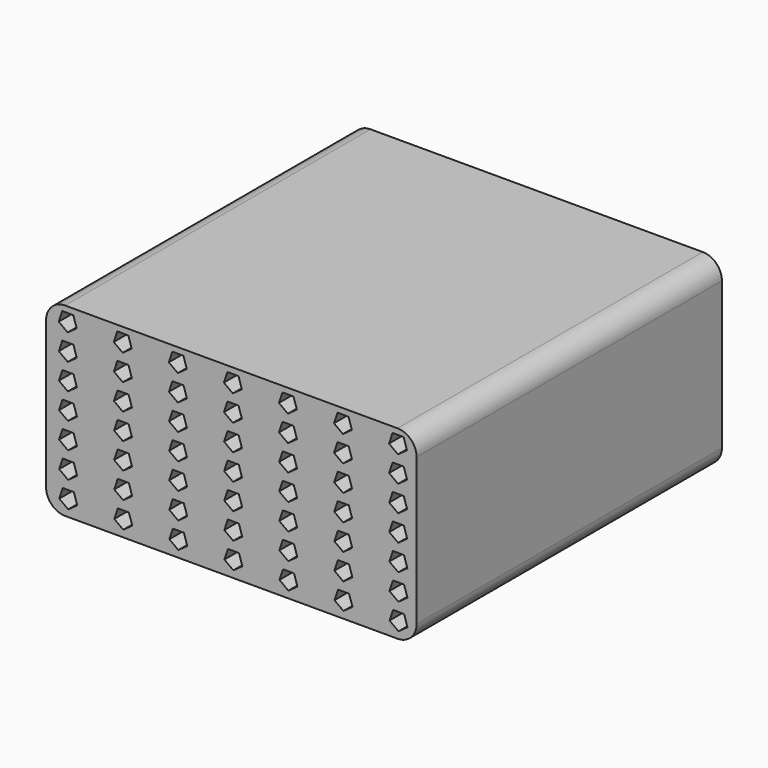
from build123d import *

# Parameters (mm, degrees)
F1_DEPTH = 127


# Not quite as in the source:
# - a feature names something its author has since deleted; it is built from what else it names


with BuildPart() as f1:
    # F0 (on Front) → F1 (new body)
    with BuildSketch(Plane.XZ):
        with BuildLine():
            ThreePointArc((61.6458, 24.4729), (59.7859280605, 28.9630280605), (55.2958, 30.8229))
            Line((55.2958, 30.8229), (-55.2958, 30.8229))
            ThreePointArc((-55.2958, 30.8229), (-59.7859280605, 28.9630280605), (-61.6458, 24.4729))
            Line((-61.6458, 24.4729), (-61.6458, -24.4729))
            ThreePointArc((-61.6458, -24.4729), (-59.7859280605, -28.9630280605), (-55.2958, -30.8229))
            Line((-55.2958, -30.8229), (55.2958, -30.8229))
            ThreePointArc((55.2958, -30.8229), (59.7859280605, -28.9630280605), (61.6458, -24.4729))
            Line((61.6458, -24.4729), (61.6458, 24.4729))
        make_face()
        Polygon((-57.2556481806, -26.3868499187), (-56.093504692, -22.8837522606), (-52.4027387491, -22.906499689), (-51.2838634405, -26.4236560311), (-54.2831264135, -28.5746307658), align=None, mode=Mode.SUBTRACT)
        Polygon((-38.9379778168, -26.3810199025), (-37.7758343281, -22.8779222443), (-34.0850683852, -22.9006696728), (-32.9661930766, -26.4178260149), (-35.9654560497, -28.5688007496), align=None, mode=Mode.SUBTRACT)
        Polygon((-57.2853185445, -17.756679935), (-56.1231750558, -14.2535822768), (-52.4324091129, -14.2763297053), (-51.3135338044, -17.7934860474), (-54.3127967774, -19.9444607821), align=None, mode=Mode.SUBTRACT)
        Polygon((-38.9676481806, -17.7508499187), (-37.805504692, -14.2477522606), (-34.1147387491, -14.270499689), (-32.9958634405, -17.7876560311), (-35.9951264135, -19.9386307658), align=None, mode=Mode.SUBTRACT)
        Polygon((-20.6203074529, -26.3751898862), (-19.4581639642, -22.8720922281), (-15.7673980213, -22.8948396565), (-14.6485227127, -26.4119959986), (-17.6477856858, -28.5629707333), align=None, mode=Mode.SUBTRACT)
        Polygon((-20.6499778168, -17.7450199025), (-19.4878343281, -14.2419222443), (-15.7970683852, -14.2646696728), (-14.6781930766, -17.7818260149), (-17.6774560497, -19.9328007496), align=None, mode=Mode.SUBTRACT)
        Polygon((-57.3149889084, -9.1265099512), (-56.1528454197, -5.6234122931), (-52.4620794768, -5.6461597215), (-51.3432041682, -9.1633160636), (-54.3424671413, -11.3142907983), align=None, mode=Mode.SUBTRACT)
        Polygon((-38.9973185445, -9.120679935), (-37.8351750558, -5.6175822768), (-34.1444091129, -5.6403297053), (-33.0255338044, -9.1574860474), (-36.0247967774, -11.3084607821), align=None, mode=Mode.SUBTRACT)
        Polygon((-20.6796481806, -9.1148499187), (-19.517504692, -5.6117522606), (-15.8267387491, -5.634499689), (-14.7078634405, -9.1516560311), (-17.7071264135, -11.3026307658), align=None, mode=Mode.SUBTRACT)
        Polygon((-2.302637089, -26.36935987), (-1.1404936004, -22.8662622118), (2.5502723426, -22.8890096402), (3.6691476511, -26.4061659823), (0.6698846781, -28.5571407171), align=None, mode=Mode.SUBTRACT)
        Polygon((16.0150332748, -26.3635298537), (17.1771767635, -22.8604321955), (20.8679427064, -22.883179624), (21.986818015, -26.4003359661), (18.987555042, -28.5513107008), align=None, mode=Mode.SUBTRACT)
        Polygon((-2.3323074529, -17.7391898862), (-1.1701639642, -14.2360922281), (2.5206019787, -14.2588396565), (3.6394772873, -17.7759959986), (0.6402143142, -19.9269707333), align=None, mode=Mode.SUBTRACT)
        Polygon((15.985362911, -17.73335987), (17.1475063996, -14.2302622118), (20.8382723426, -14.2530096402), (21.9571476511, -17.7701659823), (18.9578846781, -19.9211407171), align=None, mode=Mode.SUBTRACT)
        Polygon((34.3327036387, -26.3576998375), (35.4948471274, -22.8546021793), (39.1856130703, -22.8773496077), (40.3044883789, -26.3945059498), (37.3052254058, -28.5454806846), align=None, mode=Mode.SUBTRACT)
        Polygon((52.6503740026, -26.3518698212), (53.8125174913, -22.848772163), (57.5032834342, -22.8715195915), (58.6221587428, -26.3886759336), (55.6228957697, -28.5396506683), align=None, mode=Mode.SUBTRACT)
        Polygon((34.3030332748, -17.7275298537), (35.4651767635, -14.2244321955), (39.1559427064, -14.247179624), (40.274818015, -17.7643359661), (37.275555042, -19.9153107008), align=None, mode=Mode.SUBTRACT)
        Polygon((52.6207036387, -17.7216998375), (53.7828471274, -14.2186021793), (57.4736130703, -14.2413496077), (58.5924883789, -17.7585059498), (55.5932254058, -19.9094806846), align=None, mode=Mode.SUBTRACT)
        Polygon((-2.3619778168, -9.1090199025), (-1.1998343281, -5.6059222443), (2.4909316148, -5.6286696728), (3.6098069234, -9.1458260149), (0.6105439503, -11.2968007496), align=None, mode=Mode.SUBTRACT)
        Polygon((15.9556925471, -9.1031898862), (17.1178360358, -5.6000922281), (20.8086019787, -5.6228396565), (21.9274772873, -9.1399959986), (18.9282143142, -11.2909707333), align=None, mode=Mode.SUBTRACT)
        Polygon((34.273362911, -9.09735987), (35.4355063996, -5.5942622118), (39.1262723426, -5.6170096402), (40.2451476511, -9.1341659823), (37.2458846781, -11.2851407171), align=None, mode=Mode.SUBTRACT)
        Polygon((52.5910332748, -9.0915298537), (53.7531767635, -5.5884321955), (57.4439427064, -5.611179624), (58.562818015, -9.1283359661), (55.563555042, -11.2793107008), align=None, mode=Mode.SUBTRACT)
        Polygon((-57.3446592723, -0.4963399675), (-56.1825157836, 3.0067576907), (-52.4917498407, 2.9840102622), (-51.3728745321, -0.5331460799), (-54.3721375051, -2.6841208146), align=None, mode=Mode.SUBTRACT)
        Polygon((-39.0269889084, -0.4905099512), (-37.8648454197, 3.0125877069), (-34.1740794768, 2.9898402785), (-33.0552041682, -0.5273160636), (-36.0544671413, -2.6782907983), align=None, mode=Mode.SUBTRACT)
        Polygon((-57.3743296361, 8.1338300163), (-56.2121861475, 11.6369276744), (-52.5214202045, 11.614180246), (-51.402544896, 8.0970239039), (-54.401807869, 5.9460491692), align=None, mode=Mode.SUBTRACT)
        Polygon((-39.0566592723, 8.1396600325), (-37.8945157836, 11.6427576907), (-34.2037498407, 11.6200102622), (-33.0848745321, 8.1028539201), (-36.0841375051, 5.9518791854), align=None, mode=Mode.SUBTRACT)
        Polygon((-20.7093185445, -0.484679935), (-19.5471750558, 3.0184177232), (-15.8564091129, 2.9956702947), (-14.7375338044, -0.5214860474), (-17.7367967774, -2.6724607821), align=None, mode=Mode.SUBTRACT)
        Polygon((-20.7389889084, 8.1454900488), (-19.5768454197, 11.6485877069), (-15.8860794768, 11.6258402785), (-14.7672041682, 8.1086839364), (-17.7664671413, 5.9577092017), align=None, mode=Mode.SUBTRACT)
        Polygon((-57.404, 16.764), (-56.2418565113, 20.2670976582), (-52.5510905684, 20.2443502297), (-51.4322152598, 16.7271938876), (-54.4314782329, 14.5762191529), align=None, mode=Mode.SUBTRACT)
        Polygon((-39.0863296361, 16.7698300163), (-37.9241861475, 20.2729276744), (-34.2334202045, 20.250180246), (-33.114544896, 16.7330239039), (-36.113807869, 14.5820491692), align=None, mode=Mode.SUBTRACT)
        Polygon((-56.2715268752, 28.8972676419), (-52.5807609323, 28.8745202135), (-51.4618856237, 25.3573638714), (-54.4611485968, 23.2063891366), (-57.4336703639, 25.3941699837), align=None, mode=Mode.SUBTRACT)
        Polygon((-39.116, 25.4), (-37.9538565113, 28.9030976582), (-34.2630905684, 28.8803502297), (-33.1442152598, 25.3631938876), (-36.1434782329, 23.2122191529), align=None, mode=Mode.SUBTRACT)
        Polygon((-20.7686592723, 16.7756600325), (-19.6065157836, 20.2787576907), (-15.9157498407, 20.2560102622), (-14.7968745321, 16.7388539201), (-17.7961375051, 14.5878791854), align=None, mode=Mode.SUBTRACT)
        Polygon((-20.7983296361, 25.4058300163), (-19.6361861475, 28.9089276744), (-15.9454202045, 28.886180246), (-14.826544896, 25.3690239039), (-17.825807869, 23.2180491692), align=None, mode=Mode.SUBTRACT)
        Polygon((-2.3916481806, -0.4788499187), (-1.229504692, 3.0242477394), (2.4612612509, 3.001500311), (3.5801365595, -0.5156560311), (0.5808735865, -2.6666307658), align=None, mode=Mode.SUBTRACT)
        Polygon((15.9260221832, -0.4730199025), (17.0881656719, 3.0300777557), (20.7789316148, 3.0073303272), (21.8978069234, -0.5098260149), (18.8985439503, -2.6608007496), align=None, mode=Mode.SUBTRACT)
        Polygon((-2.4213185445, 8.151320065), (-1.2591750558, 11.6544177232), (2.4315908871, 11.6316702947), (3.5504661956, 8.1145139526), (0.5512032226, 5.9635392179), align=None, mode=Mode.SUBTRACT)
        Polygon((15.8963518194, 8.1571500813), (17.058495308, 11.6602477394), (20.7492612509, 11.637500311), (21.8681365595, 8.1203439689), (18.8688735865, 5.9693692342), align=None, mode=Mode.SUBTRACT)
        Polygon((34.2436925471, -0.4671898862), (35.4058360358, 3.0359077719), (39.0966019787, 3.0131603435), (40.2154772873, -0.5039959986), (37.2162143142, -2.6549707333), align=None, mode=Mode.SUBTRACT)
        Polygon((52.561362911, -0.46135987), (53.7235063996, 3.0417377882), (57.4142723426, 3.0189903598), (58.5331476511, -0.4981659823), (55.5338846781, -2.6491407171), align=None, mode=Mode.SUBTRACT)
        Polygon((34.2140221832, 8.1629800975), (35.3761656719, 11.6660777557), (39.0669316148, 11.6433303272), (40.1858069234, 8.1261739851), (37.1865439503, 5.9751992504), align=None, mode=Mode.SUBTRACT)
        Polygon((52.5316925471, 8.1688101138), (53.6938360358, 11.6719077719), (57.3846019787, 11.6491603435), (58.5034772873, 8.1320040014), (55.5042143142, 5.9810292667), align=None, mode=Mode.SUBTRACT)
        Polygon((-2.4509889084, 16.7814900488), (-1.2888454197, 20.2845877069), (2.4019205232, 20.2618402785), (3.5207958318, 16.7446839364), (0.5215328587, 14.5937092017), align=None, mode=Mode.SUBTRACT)
        Polygon((15.8666814555, 16.787320065), (17.0288249442, 20.2904177232), (20.7195908871, 20.2676702947), (21.8384661956, 16.7505139526), (18.8392032226, 14.5995392179), align=None, mode=Mode.SUBTRACT)
        Polygon((-2.4806592723, 25.4116600325), (-1.3185157836, 28.9147576907), (2.3722501593, 28.8920102622), (3.4911254679, 25.3748539201), (0.4918624949, 23.2238791854), align=None, mode=Mode.SUBTRACT)
        Polygon((15.8370110916, 25.4174900488), (16.9991545803, 28.9205877069), (20.6899205232, 28.8978402785), (21.8087958318, 25.3806839364), (18.8095328587, 23.2297092017), align=None, mode=Mode.SUBTRACT)
        Polygon((34.1843518194, 16.7931500813), (35.346495308, 20.2962477394), (39.0372612509, 20.273500311), (40.1561365595, 16.7563439689), (37.1568735865, 14.6053692342), align=None, mode=Mode.SUBTRACT)
        Polygon((52.5020221832, 16.7989800975), (53.6641656719, 20.3020777557), (57.3549316148, 20.2793303272), (58.4738069234, 16.7621739851), (55.4745439503, 14.6111992504), align=None, mode=Mode.SUBTRACT)
        Polygon((34.1546814555, 25.423320065), (35.3168249442, 28.9264177232), (39.0075908871, 28.9036702947), (40.1264661956, 25.3865139526), (37.1272032226, 23.2355392179), align=None, mode=Mode.SUBTRACT)
        Polygon((52.4723518194, 25.4291500813), (53.634495308, 28.9322477394), (57.3252612509, 28.909500311), (58.4441365595, 25.3923439689), (55.4448735865, 23.2413692342), align=None, mode=Mode.SUBTRACT)
    extrude(amount=F1_DEPTH)


solid = f1.part
